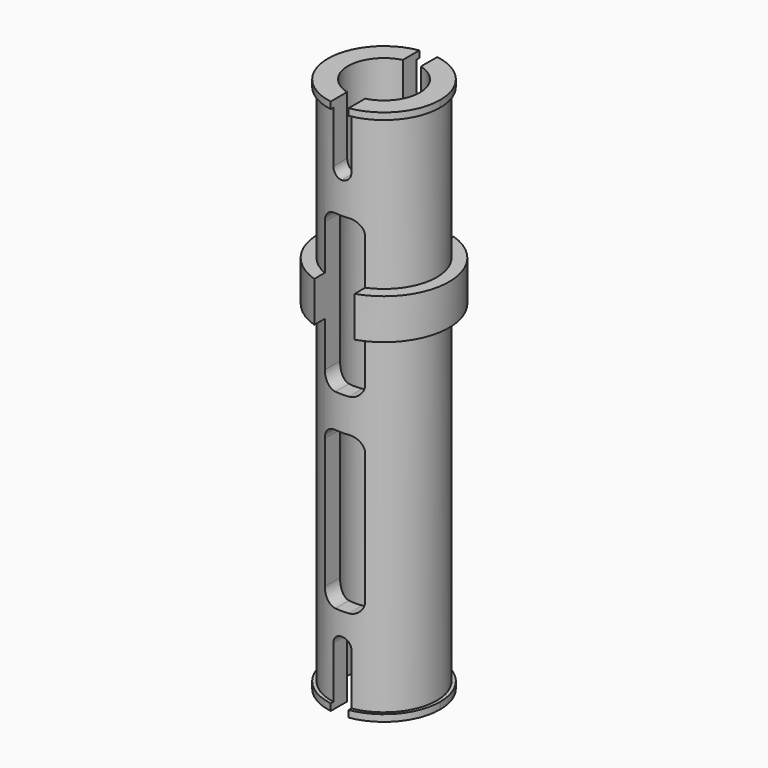
from build123d import *

# Parameters (mm, degrees)
F0_R      = 2.35
F0_R_2    = 1.6
F1_DEPTH  = 7.9
F2_DEPTH  = 16
F4_DEPTH  = 3
F6_DEPTH  = 3
F7_R      = 0.3999
F0_R_3    = 2.9
F8_DEPTH  = 0.9
F10_DEPTH = 0.3
F12_DEPTH = 0.3
F14_DEPTH = 0.3
F16_DEPTH = 0.3
F17_W     = 1.8
F17_H     = 7
F18_DEPTH = 12.5
F19_R     = 0.6


# Not quite as in the source:
# - a fillet or chamfer is up to 0.001 mm smaller than in the source, because OpenCascade refuses the exact size


with BuildPart() as f1:
    # F0 (on Top) → F1 (new body)
    with BuildSketch(Plane.XY):
        Circle(F0_R)
        Circle(F0_R_2, mode=Mode.SUBTRACT)
    extrude(amount=F1_DEPTH)

    # F0 (on Top) → F2 (join)
    with BuildSketch(Plane.XY):
        Circle(F0_R)
        Circle(F0_R_2, mode=Mode.SUBTRACT)
    extrude(amount=-F2_DEPTH)

    # F3 (on face) → F4 (cut)
    with BuildSketch(Plane.XY.offset(7.9)):
        with BuildLine():
            Line((-0.4, 2.3157072354), (-0.4, 1.6))
            Line((-0.4, 1.6), (-0.4, 1.5491933385))
            ThreePointArc((-0.4, 1.5491933385), (-0.201606868, 1.587247514), (0, 1.6))
            ThreePointArc((0, 1.6), (0.201606868, 1.587247514), (0.4, 1.5491933385))
            Line((0.4, 1.5491933385), (0.4, 1.6))
            Line((0.4, 1.6), (0.4, 2.3157072354))
            ThreePointArc((0.4, 2.3157072354), (0, 2.35), (-0.4, 2.3157072354))
        make_face()
        with BuildLine():
            Line((-0.4, -1.6), (-0.4, -2.3157072354))
            ThreePointArc((-0.4, -2.3157072354), (0, -2.35), (0.4, -2.3157072354))
            Line((0.4, -2.3157072354), (0.4, -1.6))
            Line((0.4, -1.6), (0.4, -1.5491933385))
            ThreePointArc((0.4, -1.5491933385), (0, -1.6), (-0.4, -1.5491933385))
            Line((-0.4, -1.5491933385), (-0.4, -1.6))
        make_face()
    extrude(amount=-F4_DEPTH, mode=Mode.SUBTRACT)

    # F5 (on face) → F6 (cut)
    with BuildSketch(Plane(origin=(0, 0, -16), x_dir=(1, 0, 0), z_dir=(0, 0, -1))):
        with BuildLine():
            Line((-0.4, 2.3157072354), (-0.4, 1.6))
            Line((-0.4, 1.6), (-0.4, 1.5491933385))
            ThreePointArc((-0.4, 1.5491933385), (-0.201606868, 1.587247514), (0, 1.6))
            ThreePointArc((0, 1.6), (0.201606868, 1.587247514), (0.4, 1.5491933385))
            Line((0.4, 1.5491933385), (0.4, 2.3157072354))
            ThreePointArc((0.4, 2.3157072354), (0, 2.35), (-0.4, 2.3157072354))
        make_face()
        with BuildLine():
            Line((-0.4, -1.6), (-0.4, -2.3157072354))
            ThreePointArc((-0.4, -2.3157072354), (0, -2.35), (0.4, -2.3157072354))
            Line((0.4, -2.3157072354), (0.4, -1.5491933385))
            ThreePointArc((0.4, -1.5491933385), (0, -1.6), (-0.4, -1.5491933385))
            Line((-0.4, -1.5491933385), (-0.4, -1.6))
        make_face()
    extrude(amount=-F6_DEPTH, mode=Mode.SUBTRACT)

    # F7 (radius 0.4 in the source; OpenCascade refuses exactly that, so slightly less here)
    f7_edges = [f1.edges().sort_by_distance(p)[0] for p in [
        (-0.4, -1.93245, 4.9),
        (0.4, -1.93245, 4.9),
        (0.4, 1.93245, 4.9),
        (-0.4, 1.93245, 4.9),
        (0.4, -1.93245, -13),
        (-0.4, -1.93245, -13),
        (-0.4, 1.93245, -13),
        (0.4, 1.93245, -13),
    ]]
    fillet(f7_edges, radius=F7_R)

    # F0 (on Top) → F8 (join, symmetric)
    with BuildSketch(Plane.XY):
        Circle(F0_R_3)
        Circle(F0_R, mode=Mode.SUBTRACT)
    extrude(amount=F8_DEPTH, both=True)

    # F9 (on face) → F10 (join)
    with BuildSketch(Plane(origin=(0, 0, -16), x_dir=(1, 0, 0), z_dir=(0, 0, -1))):
        with BuildLine():
            ThreePointArc((-0.4, -2.3157072354), (-2.35, 0), (-0.4, 2.3157072354))
            Line((-0.4, 2.3157072354), (-0.4, 2.4677925359))
            ThreePointArc((-0.4, 2.4677925359), (-2.5, 0), (-0.4, -2.4677925359))
            Line((-0.4, -2.4677925359), (-0.4, -2.3157072354))
        make_face()
    extrude(amount=-F10_DEPTH)

    # F11 (on face) → F12 (join)
    with BuildSketch(Plane(origin=(0, 0, -16), x_dir=(1, 0, 0), z_dir=(0, 0, -1))):
        with BuildLine():
            ThreePointArc((0.4, -2.4677925359), (1.9039432765, -1.6201851746), (2.5, 0))
            ThreePointArc((2.5, 0), (1.9039432765, 1.6201851746), (0.4, 2.4677925359))
            Line((0.4, 2.4677925359), (0.4, 2.3157072354))
            ThreePointArc((0.4, 2.3157072354), (1.7975678012, 1.5136875503), (2.35, 0))
            ThreePointArc((2.35, 0), (1.7975678012, -1.5136875503), (0.4, -2.3157072354))
            Line((0.4, -2.3157072354), (0.4, -2.4677925359))
        make_face()
    extrude(amount=-F12_DEPTH)

    # F13 (on face) → F14 (join)
    with BuildSketch(Plane.XY.offset(7.9)):
        with BuildLine():
            Line((-0.4, 2.3157072354), (-0.4, 2.4677925359))
            ThreePointArc((-0.4, 2.4677925359), (-2.5, 0), (-0.4, -2.4677925359))
            Line((-0.4, -2.4677925359), (-0.4, -2.3157072354))
            ThreePointArc((-0.4, -2.3157072354), (-2.35, 0), (-0.4, 2.3157072354))
        make_face()
    extrude(amount=-F14_DEPTH)

    # F15 (on face) → F16 (join)
    with BuildSketch(Plane.XY.offset(7.9)):
        with BuildLine():
            ThreePointArc((0.4, -2.4677925359), (1.9039432765, -1.6201851746), (2.5, 0))
            ThreePointArc((2.5, 0), (1.9039432765, 1.6201851746), (0.4, 2.4677925359))
            Line((0.4, 2.4677925359), (0.4, 2.3157072354))
            ThreePointArc((0.4, 2.3157072354), (1.7975678012, 1.5136875503), (2.35, 0))
            ThreePointArc((2.35, 0), (1.7975678012, -1.5136875503), (0.4, -2.3157072354))
            Line((0.4, -2.3157072354), (0.4, -2.4677925359))
        make_face()
    extrude(amount=-F16_DEPTH)

    # F17 (on Front) → F18 (cut, symmetric)
    with BuildSketch(Plane.XZ):
        Polygon((0.9, -3.5), (0.9, 0), (0.9, 3.5), (-0.9, 3.5), (-0.9, -3.5), align=None)
        with Locations((0, -8.5)):
            Rectangle(F17_W, F17_H)
    extrude(amount=F18_DEPTH, both=True, mode=Mode.SUBTRACT)

    # F19
    f19_edges = [f1.edges().sort_by_distance(p)[0] for p in [
        (-0.9, -1.746852, 3.5),
        (-0.9, 1.746852, 3.5),
        (0.9, -1.746852, 3.5),
        (0.9, 1.746852, 3.5),
        (0.9, -1.746852, -3.5),
        (0.9, 1.746852, -3.5),
        (-0.9, -1.746852, -3.5),
        (-0.9, 1.746852, -3.5),
        (0.9, -1.746852, -5),
        (0.9, 1.746852, -5),
        (-0.9, -1.746852, -5),
        (-0.9, 1.746852, -5),
        (0.9, -1.746852, -12),
        (0.9, 1.746852, -12),
        (-0.9, -1.746852, -12),
        (-0.9, 1.746852, -12),
    ]]
    fillet(f19_edges, radius=F19_R)


solid = f1.part
